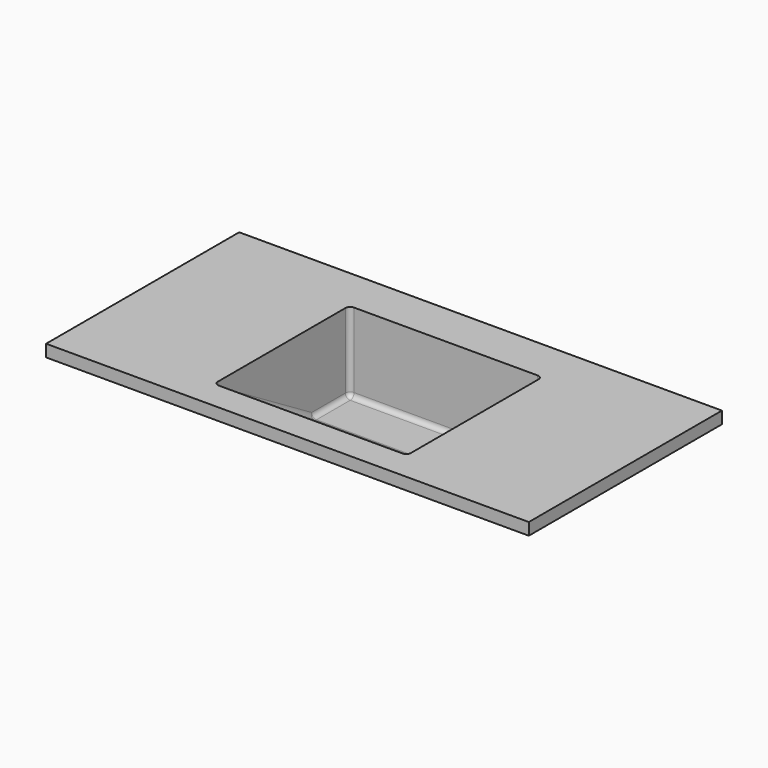
from build123d import *

# Parameters (mm, degrees)
F0_W      = 1000
F0_H      = 500
F1_DEPTH  = 25
F2_W      = 400
F2_H      = 350
F3_DEPTH  = 25
F4_W      = 450
F4_H      = 25
F5_DEPTH  = 165
F6_W      = 450
F6_H      = 25
F7_DEPTH  = 100
F9_DEPTH  = 25
F10_W     = 450
F10_H     = 320.7023542165
F11_DEPTH = 21.4373231428
F12_R     = 10


# Not quite as in the source:
# - a pattern or mirror of a feature is missing from the dataset's text; its kind, count and spacing are read off the source's solid


with BuildPart() as f1:
    # F0 (on Top) → F1 (new body)
    with BuildSketch(Plane.XY):
        Rectangle(F0_W, F0_H)
    extrude(amount=F1_DEPTH)

    # F2 (on face) → F3 (cut, through all)
    with BuildSketch(Plane.XY.offset(25)):
        with Locations((0, -15)):
            Rectangle(F2_W, F2_H)
    extrude(amount=-F3_DEPTH, mode=Mode.SUBTRACT)

    # F4 (on face) → F5 (join)
    with BuildSketch(Plane(origin=(0, 0, 0), x_dir=(1, 0, 0), z_dir=(0, 0, -1))):
        with Locations((0, -172.5)):
            Rectangle(F4_W, F4_H)
    extrude(amount=F5_DEPTH)

    # F6 (on face) → F7 (join)
    with BuildSketch(Plane.XZ.offset(-160)):
        with Locations((0, -152.5)):
            Rectangle(F6_W, F6_H)
    extrude(amount=F7_DEPTH)

    # F8 (on face) → F9 (join)
    with BuildSketch(Plane(origin=(-225, 0, 0), x_dir=(0, -1, 0), z_dir=(-1, 0, 0))):
        Polygon((215, 0), (-185, 0), (-185, -165), (-60, -165), align=None)
    f9 = extrude(amount=-F9_DEPTH)

    # F9_copies: F9 across plane
    add(f9.mirror(Plane(origin=(0, 0, 0), x_dir=(0, 0, 1), z_dir=(1, 0, 0))))

    # F10 (on face) → F11 (join, through all)
    with BuildSketch(Plane(origin=(0, -56.9117647059, -94.8529411765), x_dir=(1, 0, 0), z_dir=(0, -0.5144957554, -0.8574929257))):
        with Locations((0, 24.00980192)):
            Rectangle(F10_W, F10_H)
    extrude(amount=-F11_DEPTH)

    # F12
    f12_edges = [f1.edges().sort_by_distance(p)[0] for p in [
        (0, 160, -140),
        (-200, 110, -140),
        (-200, 160, -57.5),
        (0, 60, -140),
        (-200, -65, -65),
        (-200, -190, 17.5),
        (200, -190, 17.5),
        (0, -190, 10),
        (200, 160, -57.5),
        (200, 110, -140),
        (200, -65, -65),
    ]]
    fillet(f12_edges, radius=F12_R)


solid = f1.part
